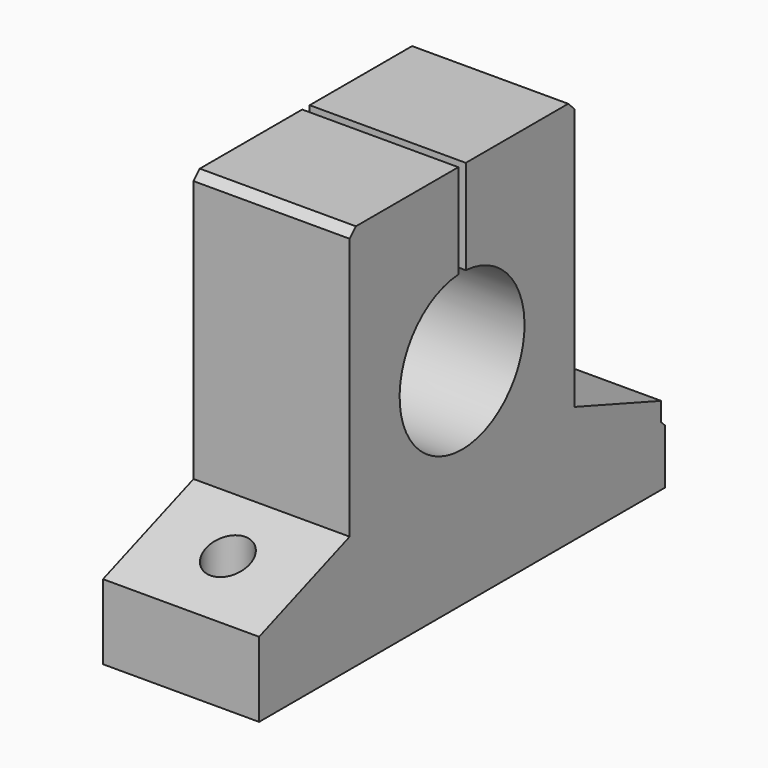
from build123d import *

# Parameters (mm, degrees)
F1_DEPTH = 12.7
F2_R     = 3.556
F3_DEPTH = 62.993


# Not quite as in the source:
# - ends of sketch curves that miss each other by under 0.0002 mm in the source are joined


with BuildPart() as f1:
    # F0 (on Right) → F1 (new body, symmetric)
    with BuildSketch(Plane.YZ):
        with BuildLine():
            Line((0.762, 33.02), (0.762, 17.6402746))
            ThreePointArc((0.762, 17.6402746), (0, -7.73684), (-0.7620002868, 17.6402793716))
            Line((-0.7620002868, 17.6402793716), (-0.762, 33.02))
            Line((-0.762, 33.02), (-21.59, 33.02))
            Line((-21.59, 33.02), (-22.86, 31.75))
            Line((-22.86, 31.75), (-22.86, -10.922))
            Line((-22.86, -10.922), (-41.275, -17.78))
            Line((-41.275, -17.78), (-41.275, -29.972))
            Line((-41.275, -29.972), (41.275, -29.972))
            Line((41.275, -29.972), (41.275, -21.0566))
            Line((41.275, -21.0566), (40.4876, -20.2692))
            Line((40.4876, -20.2692), (40.4876, -17.2175678))
            Line((40.4876, -17.2175678), (22.86, -10.922))
            Line((22.86, -10.922), (22.86, 31.75))
            Line((22.86, 31.75), (21.59, 33.02))
            Line((21.59, 33.02), (0.762, 33.02))
        make_face()
    extrude(amount=F1_DEPTH, both=True)

    # F2 (on face) → F3 (cut, through all)
    with BuildSketch(Plane(origin=(0, 0, -29.972), x_dir=(1, 0, 0), z_dir=(0, 0, -1))):
        with Locations((0, 31.75)):
            Circle(F2_R)
        with Locations((0, -31.75)):
            Circle(F2_R)
    extrude(amount=-F3_DEPTH, mode=Mode.SUBTRACT)


solid = f1.part
